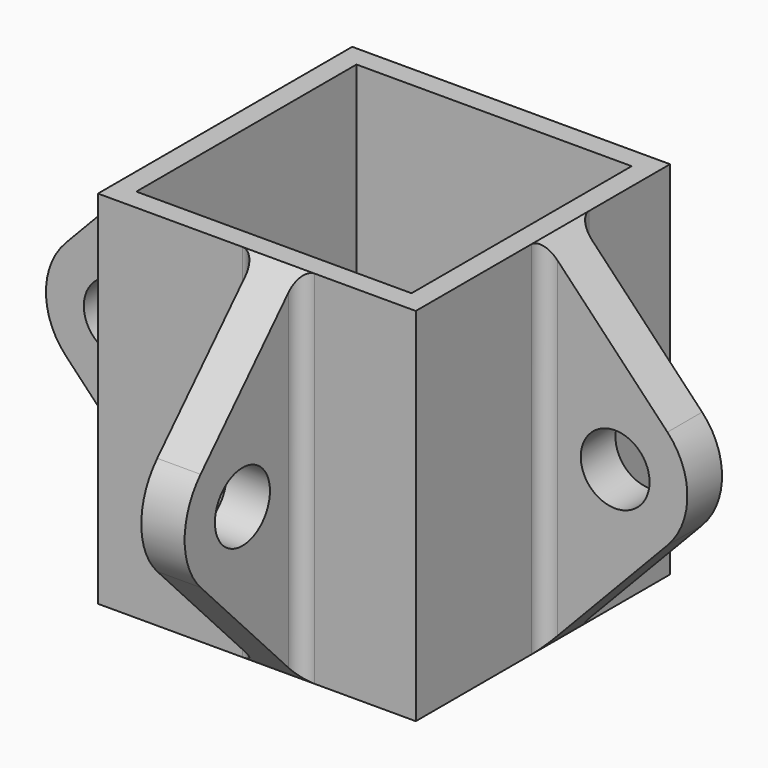
from build123d import *

# Parameters (mm, degrees)
F0_W     = 22
F0_H     = 22
F0_W_2   = 19.05
F0_H_2   = 19.05
F1_DEPTH = 12.5
F2_R     = 2.38125
F3_DEPTH = 3
F4_R     = 2.38125
F5_DEPTH = 3
F6_R     = 2.38125
F7_DEPTH = 3
F8_R     = 2.4003
F9_DEPTH = 3
F10_R    = 1


# Not quite as in the source:
# - a feature names something its author has since deleted; it is built from what else it names


with BuildPart() as f1:
    # F0 (on Top) → F1 (new body, symmetric)
    with BuildSketch(Plane.XY):
        Rectangle(F0_W, F0_H)
        Rectangle(F0_W_2, F0_H_2, mode=Mode.SUBTRACT)
    extrude(amount=F1_DEPTH, both=True)

    # F2 (on Front) → F3 (join)
    with BuildSketch(Plane.XZ):
        with BuildLine():
            Line((-11, -12.5), (-11, 12.5))
            Line((-11, 12.5), (-19.6206896552, 3.4482758621))
            ThreePointArc((-19.6206896552, 3.4482758621), (-21, 0), (-19.6206896552, -3.4482758621))
            Line((-19.6206896552, -3.4482758621), (-11, -12.5))
        make_face()
        with Locations((-16, 0)):
            Circle(F2_R, mode=Mode.SUBTRACT)
    extrude(amount=F3_DEPTH)

    # F4 (on Right) → F5 (join)
    with BuildSketch(Plane.YZ):
        with BuildLine():
            Line((-11, 12.5), (-19.6206896552, 3.4482758621))
            ThreePointArc((-19.6206896552, 3.4482758621), (-21, 0), (-19.6206896552, -3.4482758621))
            Line((-19.6206896552, -3.4482758621), (-11, -12.5))
            Line((-11, -12.5), (-11, 12.5))
        make_face()
        with Locations((-16, 0)):
            Circle(F4_R, mode=Mode.SUBTRACT)
    extrude(amount=F5_DEPTH)

    # F6 (on Front) → F7 (join)
    with BuildSketch(Plane.XZ):
        with BuildLine():
            Line((11, -12.5), (19.6206896552, -3.4482758621))
            ThreePointArc((19.6206896552, -3.4482758621), (21, 0), (19.6206896552, 3.4482758621))
            Line((19.6206896552, 3.4482758621), (11, 12.5))
            Line((11, 12.5), (11, -12.5))
        make_face()
        with Locations((16, 0)):
            Circle(F6_R, mode=Mode.SUBTRACT)
    extrude(amount=-F7_DEPTH)

    # F8 (on Right) → F9 (join)
    with BuildSketch(Plane.YZ):
        with BuildLine():
            ThreePointArc((19.6206896552, -3.4482758621), (21, 0), (19.6206896552, 3.4482758621))
            Line((19.6206896552, 3.4482758621), (11, 12.5))
            Line((11, 12.5), (11, -12.5))
            Line((11, -12.5), (19.6206896552, -3.4482758621))
        make_face()
        with Locations((16, 0)):
            Circle(F8_R, mode=Mode.SUBTRACT)
    extrude(amount=-F9_DEPTH)

    # F10
    f10_edges = [f1.edges().sort_by_distance(p)[0] for p in [
        (-11, -3, 0),
        (0, -11, 0),
        (3, -11, 0),
        (-11, 0, 0),
        (11, 0, 0),
        (11, 3, 0),
        (0, 11, 0),
        (-3, 11, 0),
    ]]
    fillet(f10_edges, radius=F10_R)


solid = f1.part
